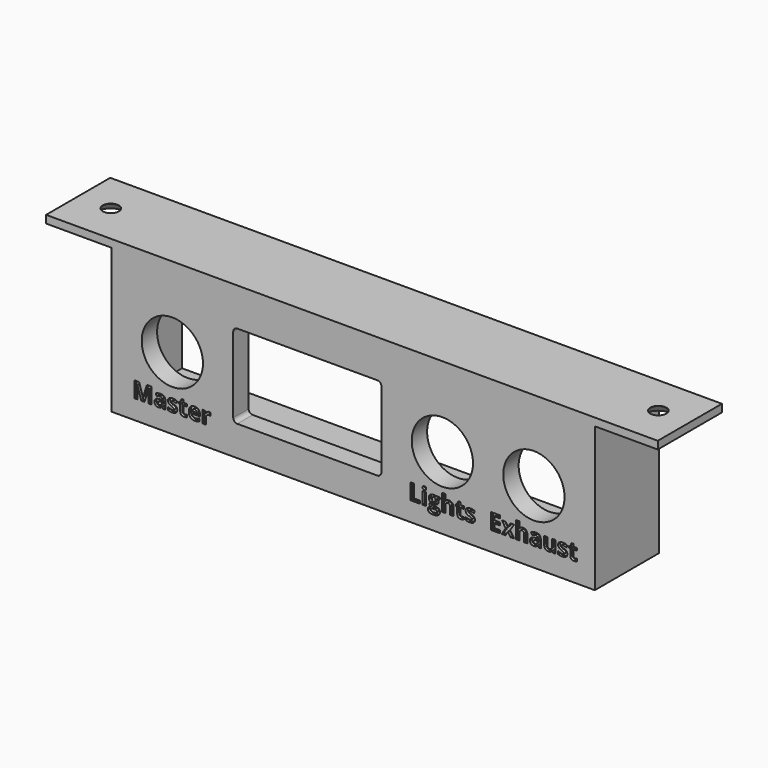
from build123d import *

# Parameters (mm, degrees)
F0_W           = 150.7
F0_H           = 45
F0_R           = 9.55
F1_DEPTH       = 6
F2_DEPTH       = 25
F4_DEPTH       = 25
F6_D           = 5.0546
F6_CSINK_D     = 9.1186
F6_CSINK_ANGLE = 82
F7_TEXT_SIZE   = 6.9444444444
F8_DEPTH       = 0.8


# Not quite as in the source:
# - Text() gives the source's letters only with a copy of the font that has no kerning and outlines rounded to 1/6400 em; it was checked with that copy


with BuildPart() as f1:
    # F0 (on Front) → F1 (new body)
    with BuildSketch(Plane.XZ):
        with Locations((0.37, 0)):
            Rectangle(F0_W, F0_H)
        with Locations((-55.99, -0.0025)):
            Circle(F0_R, mode=Mode.SUBTRACT)
        with BuildLine():
            Line((7.93, -13.0735), (-35.73, -13.0735))
            ThreePointArc((-35.73, -13.0735), (-36.6280256121, -12.7015256121), (-37, -11.8035))
            Line((-37, -11.8035), (-37, 11.7985))
            ThreePointArc((-37, 11.7985), (-36.6280256121, 12.6965256121), (-35.73, 13.0685))
            Line((-35.73, 13.0685), (7.93, 13.0685))
            ThreePointArc((7.93, 13.0685), (8.8280256121, 12.6965256121), (9.2, 11.7985))
            Line((9.2, 11.7985), (9.2, -11.8035))
            ThreePointArc((9.2, -11.8035), (8.8280256121, -12.7015256121), (7.93, -13.0735))
        make_face(mode=Mode.SUBTRACT)
        with Locations((28.19, -0.005)):
            Circle(F0_R, mode=Mode.SUBTRACT)
        with Locations((56.73, -0.005)):
            Circle(F0_R, mode=Mode.SUBTRACT)
    extrude(amount=-F1_DEPTH)

    # F0 (on Front) → F2 (join)
    with BuildSketch(Plane.XZ):
        Polygon((-95.3514990211, 22.5), (-74.98, 22.5), (75.72, 22.5), (95.3515009789, 22.5), (95.3515009789, 24.9), (-95.3514990211, 24.9), align=None)
    extrude(amount=-F2_DEPTH)

    # F3 (on Front) → F4 (join)
    with BuildSketch(Plane.XZ):
        Polygon((-74.98, 22.5), (-74.98, -22.5), (75.72, -22.5), (75.72, 22.5), (72.95, 22.5), (72.95, 20.0945567632), (72.95, -20.0945567632), (-72.95, -20.0945567632), (-72.95, 20.0945567632), (-72.95, 22.5), align=None)
    extrude(amount=-F4_DEPTH)

    # F6 (through all)
    with Locations(Plane(origin=(0, 0, 22.5), x_dir=(1, 0, 0), z_dir=(0, 0, -1))):
        with Locations((85.5357504895, -12.5), (-85.1657495105, -12.5)):
            CounterSinkHole(F6_D / 2, F6_CSINK_D / 2, counter_sink_angle=F6_CSINK_ANGLE)

    # F7 (on face) → F8 (cut)
    with BuildSketch(Plane.XZ):
        with Locations((42.7435815972, -16.4999999106)):
            Text('Exhaust', F7_TEXT_SIZE, font='Open Sans', font_style=FontStyle.BOLD, text_align=(TextAlign.LEFT, TextAlign.BOTTOM))
        with Locations((17.6116371528, -16.4999999106)):
            Text('Lights', F7_TEXT_SIZE, font='Open Sans', font_style=FontStyle.BOLD, text_align=(TextAlign.LEFT, TextAlign.BOTTOM))
        with Locations((-68.3844401042, -16.4999999106)):
            Text('Master', F7_TEXT_SIZE, font='Open Sans', font_style=FontStyle.BOLD, text_align=(TextAlign.LEFT, TextAlign.BOTTOM))
    extrude(amount=-F8_DEPTH, mode=Mode.SUBTRACT)


solid = f1.part
